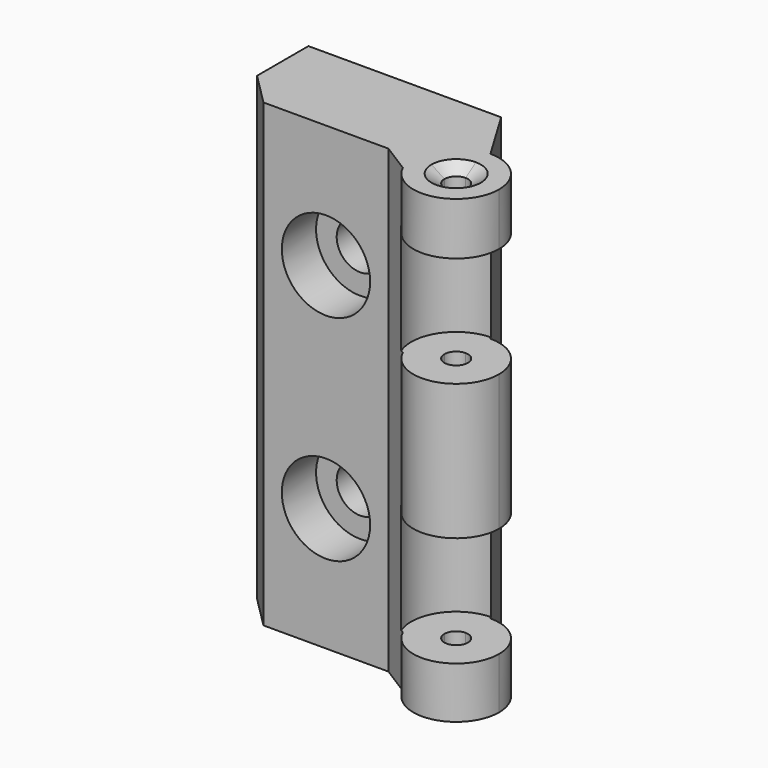
from build123d import *

# Parameters (mm, degrees)
F1_DEPTH       = 43
F2_T1_DEPTH    = 43
F2_T3_DEPTH    = 58.4300979278
F4_D           = 4.4
F4_CBORE_D     = 8.25
F4_CBORE_DEPTH = 4
F5_SIZE2       = 4.99999
F5_SIZE        = 2.99999
F7_START       = 4.8
F6_R           = 4.2
F7_DEPTH       = 10.3
F8_START       = 27.8
F8_DEPTH       = 10.3
F9_SIZE2       = 1.2
F9_SIZE        = 0.8


# Not quite as in the source:
# - a fillet or chamfer that OpenCascade refuses, or shapes differently, is made with other operations: its cross-section is extruded or revolved along the edge and cut away or added
# - a fillet or chamfer is up to 0.001 mm smaller than in the source, because OpenCascade refuses the exact size


with BuildPart() as f1:
    # F0 (on Top) → F1 (new body)
    with BuildSketch(Plane.XY):
        with BuildLine():
            Line((-10.5, -4.5), (6.5, -4.5))
            ThreePointArc((6.5, -4.5), (7.6715728753, -1.6715728753), (10.5, -0.5))
            Line((10.5, -0.5), (10.5, 4.5))
            Line((10.5, 4.5), (-10.5, 4.5))
            Line((-10.5, 4.5), (-10.5, -4.5))
        make_face()
        with BuildLine():
            Line((6.5, -4.5), (9.4, -4.5))
            ThreePointArc((9.4, -4.5), (9.7221825407, -3.7221825407), (10.5, -3.4))
            Line((10.5, -3.4), (10.5, -0.5))
            ThreePointArc((10.5, -0.5), (7.6715728753, -1.6715728753), (6.5, -4.5))
        make_face()
        with BuildLine():
            ThreePointArc((11.6, -4.5), (10.5, -5.6), (9.4, -4.5))
            Line((9.4, -4.5), (6.5, -4.5))
            ThreePointArc((6.5, -4.5), (10.5, -8.5), (14.5, -4.5))
            ThreePointArc((14.5, -4.5), (13.3284271247, -1.6715728753), (10.5, -0.5))
            Line((10.5, -0.5), (10.5, -3.4))
            ThreePointArc((10.5, -3.4), (11.2778174593, -3.7221825407), (11.6, -4.5))
        make_face()
    extrude(amount=F1_DEPTH)

    # F2: chamfer of 3 on 2 edges, made by hand

    # F2_s2 → F2_t1 (join)
    with BuildSketch(Plane.XY):
        with BuildLine():
            Line((4.1754446797, -4.5), (6.8859683884, -6.2142857143))
            ThreePointArc((6.8859683884, -6.2142857143), (6.6075772395, -5.4214364079), (6.5, -4.5))
            Line((6.5, -4.5), (4.1754446797, -4.5))
        make_face()
    extrude(amount=F2_T1_DEPTH)

    # F2_s4 → F2_t3 (cut)
    with BuildSketch(Plane.XY.offset(-7.7150489639)):
        Polygon((-7.5, -4.5), (-10.5, -1.5), (-10.5, -4.5), align=None)
    extrude(amount=F2_T3_DEPTH, mode=Mode.SUBTRACT)

    # F4 (through all)
    with Locations(Plane.XZ.offset(4.5)):
        with Locations((-1.6622776602, 31.5), (-1.6622776602, 11.5)):
            CounterBoreHole(F4_D / 2, F4_CBORE_D / 2, F4_CBORE_DEPTH)

    # F5 (size 3 and 5 in the source; OpenCascade refuses exactly that, so slightly less here)
    f5_edges = [f1.edges().sort_by_distance(p)[0] for p in [
        (10.5, 4.5, 21.5),
    ]]
    f5_side = f1.faces().sort_by_distance((0.057932, 4.5, 21.5))[0]
    chamfer(f5_edges, length=F5_SIZE, length2=F5_SIZE2, reference=f5_side)

    # F6 (on face) → F7 (cut)
    with BuildSketch(Plane.XY.offset(F7_START)):
        with Locations((10.5, -4.5)):
            Circle(F6_R)
    extrude(amount=F7_DEPTH, mode=Mode.SUBTRACT)

    # F6 (on face) → F8 (cut)
    with BuildSketch(Plane.XY.offset(F8_START)):
        with Locations((10.5, -4.5)):
            Circle(F6_R)
    extrude(amount=F8_DEPTH, mode=Mode.SUBTRACT)

    # F9
    f9_edges = [f1.edges().sort_by_distance(p)[0] for p in [
        (10.5, -5.6, 43),
    ]]
    f9_side = f1.faces().sort_by_distance((10.5, -5.6, 40.55))[0]
    chamfer(f9_edges, length=F9_SIZE, length2=F9_SIZE2, reference=f9_side)


solid = f1.part
